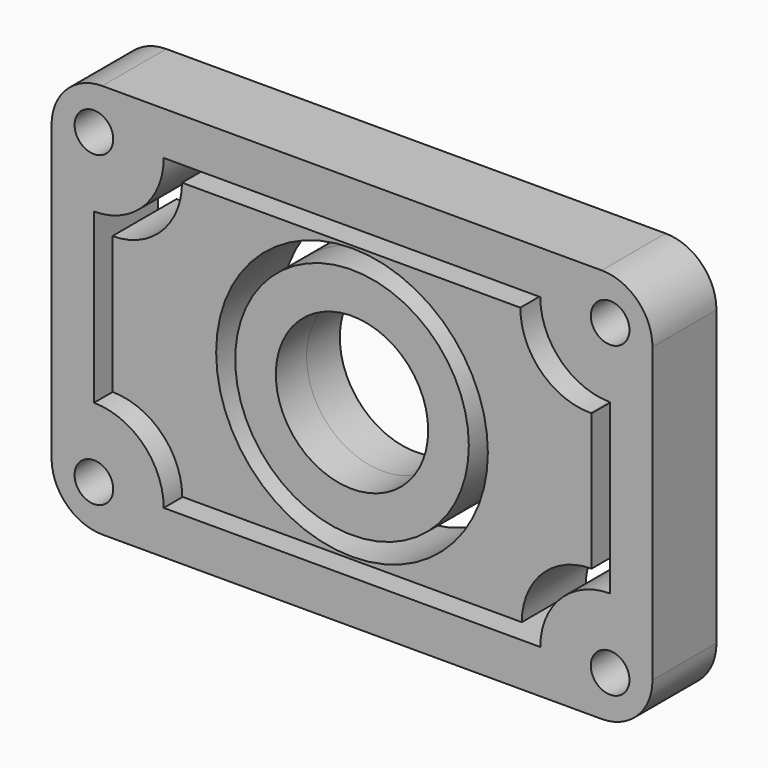
from build123d import *

# Parameters (mm, degrees)
F0_R     = 16.985
F1_DEPTH = 10
F0_R_2   = 14.605
F0_R_3   = 9.525
F2_DEPTH = 4.8
F0_R_4   = 2.415
F3_DEPTH = 10


# Not quite as in the source:
# - ends of sketch curves that miss each other by under 0.0002 mm in the source are joined


with BuildPart() as f1:
    # F0 (on Front) → F1 (new body)
    with BuildSketch(Plane.XZ):
        with BuildLine():
            Line((-21.2260876428, -17.2796698886), (21.2260876428, -17.2796698886))
            ThreePointArc((21.2260876428, -17.2796698886), (23.783045443, -11.1066276889), (29.9560876428, -8.5496698886))
            Line((29.9560876428, -8.5496698886), (29.9560876428, 8.5496698886))
            Line((29.9560876428, 8.5496698886), (29.7725021094, 8.5496698886))
            ThreePointArc((29.7725021094, 8.5496698886), (23.5994599096, 11.1066276889), (21.0425021094, 17.2796698886))
            Line((21.0425021094, 17.2796698886), (-21.2514177542, 17.2796698886))
            ThreePointArc((-21.2514177542, 17.2796698886), (-23.8009565366, 11.1245387824), (-29.9560876428, 8.575))
            Line((-29.9560876428, 8.575), (-29.9560876428, -8.575))
            ThreePointArc((-29.9560876428, -8.575), (-23.7920074576, -11.1230087778), (-21.2260876428, -17.2796698886))
        make_face()
        Circle(F0_R, mode=Mode.SUBTRACT)
    extrude(amount=F1_DEPTH)


with BuildPart() as f1b:
    # F0 (on Front) → F1, piece 2 (new body)
    with BuildSketch(Plane.XZ):
        Circle(F0_R_2)
        Circle(F0_R_3, mode=Mode.SUBTRACT)
    extrude(amount=F1_DEPTH)


with BuildPart() as f2:
    # F2 (new): a face of the model
    f2_faces = [f1b.part.faces().sort_by_distance(p)[0] for p in [
        (-14.1919082184, -10, 0),
    ]]
    extrude(f2_faces, amount=-F2_DEPTH)


with BuildPart() as f3:
    # F0 (on Front) → F3 (new body)
    with BuildSketch(Plane.XZ):
        with BuildLine():
            Line((31.2130296767, 24.6882159263), (-31.2130296767, 24.6882159263))
            ThreePointArc((-31.2130296767, 24.6882159263), (-35.7031577372, 22.8283439868), (-37.5630296767, 18.3382159263))
            Line((-37.5630296767, 18.3382159263), (-37.5630296767, -18.3382159263))
            ThreePointArc((-37.5630296767, -18.3382159263), (-35.7031577372, -22.8283439868), (-31.2130296767, -24.6882159263))
            Line((-31.2130296767, -24.6882159263), (31.2130296767, -24.6882159263))
            ThreePointArc((31.2130296767, -24.6882159263), (35.7031577372, -22.8283439868), (37.5630296767, -18.3382159263))
            Line((37.5630296767, -18.3382159263), (37.5630296767, 18.3382159263))
            ThreePointArc((37.5630296767, 18.3382159263), (35.7031577372, 22.8283439868), (31.2130296767, 24.6882159263))
        make_face()
        with Locations((-32.2686284781, -19.2572141065)):
            Circle(F0_R_4, mode=Mode.SUBTRACT)
        with Locations((32.2686284781, -19.2572141065)):
            Circle(F0_R_4, mode=Mode.SUBTRACT)
        with Locations((-32.2686284781, 19.2572141065)):
            Circle(F0_R_4, mode=Mode.SUBTRACT)
        with BuildLine():
            ThreePointArc((32.2686284781, -10.5272141065), (26.0955862783, -13.0841719068), (23.5386284781, -19.2572141065))
            Line((23.5386284781, -19.2572141065), (-23.5386284781, -19.2572141065))
            ThreePointArc((-23.5386284781, -19.2572141065), (-26.0955862783, -13.0841719068), (-32.2686284781, -10.5272141065))
            Line((-32.2686284781, -10.5272141065), (-32.2686284781, 10.5272141065))
            ThreePointArc((-32.2686284781, 10.5272141065), (-26.0955862783, 13.0841719068), (-23.5386284781, 19.2572141065))
            Line((-23.5386284781, 19.2572141065), (23.5386284781, 19.2572141065))
            ThreePointArc((23.5386284781, 19.2572141065), (26.0955862783, 13.0841719068), (32.2686284781, 10.5272141065))
            Line((32.2686284781, 10.5272141065), (32.2686284781, -10.5272141065))
        make_face(mode=Mode.SUBTRACT)
        with Locations((32.2686284781, 19.2572141065)):
            Circle(F0_R_4, mode=Mode.SUBTRACT)
    extrude(amount=F3_DEPTH)


solid = Compound([f1.part, f1b.part, f2.part, f3.part])
